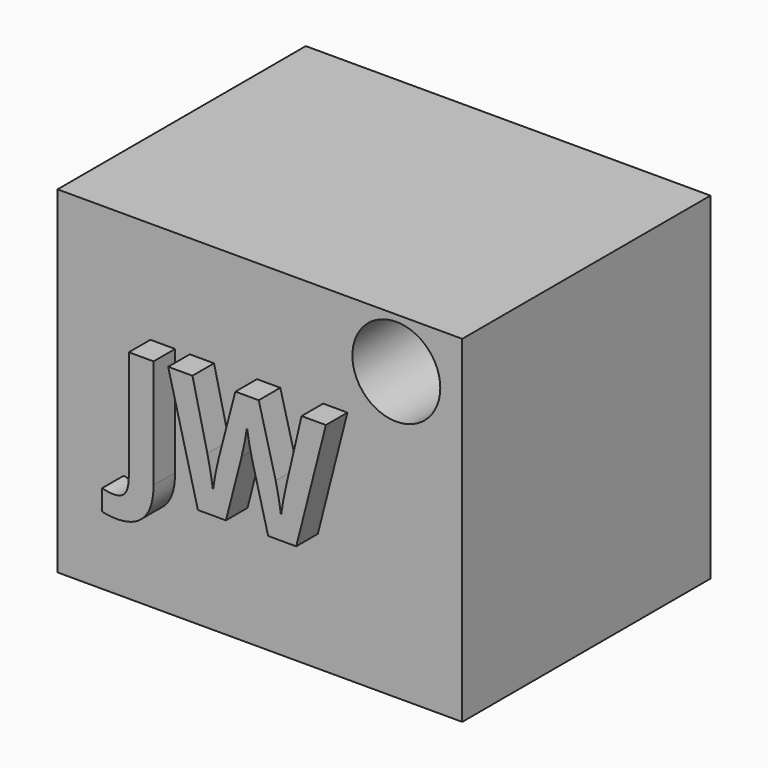
from build123d import *

# Parameters (mm, degrees)
F0_W         = 30
F0_H         = 25
F2_DEPTH     = 23
F1_TEXT_SIZE = 12.0913894433
F3_DEPTH     = 2
F4_R         = 3.2586993179
F5_DEPTH     = 42.3


# Not quite as in the source:
# - Text() gives the source's letters only with a copy of the font that has no kerning and outlines rounded to 1/6400 em; it was checked with that copy


with BuildPart() as f2:
    # F0 (on Front) → F2 (new body)
    with BuildSketch(Plane.XZ):
        Rectangle(F0_W, F0_H)
    extrude(amount=-F2_DEPTH)

    # F1 (on face) → F3 (join)
    with BuildSketch(Plane.XZ):
        with Locations((-9.2025632039, -3.7107476965)):
            Text('JW', F1_TEXT_SIZE, font='Open Sans', font_style=FontStyle.BOLD, text_align=(TextAlign.LEFT, TextAlign.BOTTOM))
    extrude(amount=F3_DEPTH)

    # F4 (on face) → F5 (cut)
    with BuildSketch(Plane.XZ):
        with Locations((10.1134423167, 8.7649831548)):
            Circle(F4_R)
    extrude(amount=-F5_DEPTH, mode=Mode.SUBTRACT)


solid = f2.part
